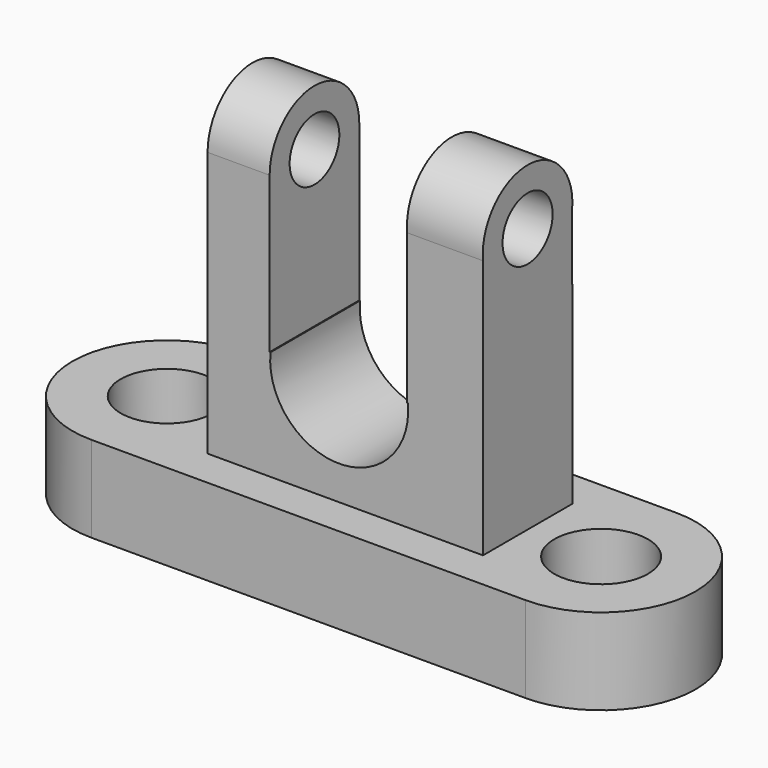
from build123d import *

# Parameters (mm, degrees)
F0_R     = 13.6198201134
F0_R_2   = 13.8204624453
F1_DEPTH = 25.4
F3_DEPTH = 16.51
F4_R     = 9.1529854274
F5_DEPTH = 18.288
F6_R     = 9.2248596532
F7_DEPTH = 22.352


# Not quite as in the source:
# - a feature names something its author has since deleted; it is built from what else it names


with BuildPart() as f1:
    # F0 (on Top) → F1 (new body)
    with BuildSketch(Plane.XY):
        with BuildLine():
            Line((-63.97113204, -27.8375800699), (63.97113204, -27.8375800699))
            ThreePointArc((63.97113204, -27.8375800699), (91.8087121099, 0), (63.97113204, 27.8375800699))
            Line((63.97113204, 27.8375800699), (-63.97113204, 27.8375800699))
            ThreePointArc((-63.97113204, 27.8375800699), (-91.8087121099, 0), (-63.97113204, -27.8375800699))
        make_face()
        with Locations((-63.97113204, 0)):
            Circle(F0_R, mode=Mode.SUBTRACT)
        with Locations((63.97113204, 0)):
            Circle(F0_R_2, mode=Mode.SUBTRACT)
    extrude(amount=-F1_DEPTH)


with BuildPart() as f3:
    # F2 (on Front) → F3 (new body, symmetric)
    with BuildSketch(Plane.XZ):
        with BuildLine():
            Line((-38.7753397226, 32.2974100709), (-38.7753397226, 0))
            Line((-38.7753397226, 0), (42.3823483288, 0))
            Line((42.3823483288, 0), (42.3823483288, 32.2974100709))
            Line((42.3823483288, 32.2974100709), (20.2484317124, 32.2974100709))
            ThreePointArc((20.2484317124, 32.2974100709), (0, 10.0047543374), (-20.2484317124, 32.2974100709))
            Line((-20.2484317124, 32.2974100709), (-38.7753397226, 32.2974100709))
        make_face()
    extrude(amount=F3_DEPTH, both=True)

    # F4 (on face) → F5 (join)
    with BuildSketch(Plane(origin=(-38.7753397226, 0, 0), x_dir=(0, -1, 0), z_dir=(-1, 0, 0))):
        with BuildLine():
            Line((-16.51, 78.1664475799), (-16.51, 56.965649128))
            Line((-16.51, 56.965649128), (-16.51, 32.2974100709))
            Line((-16.51, 32.2974100709), (16.51, 32.2974100709))
            Line((16.51, 32.2974100709), (16.51, 56.965649128))
            Line((16.51, 56.965649128), (16.51, 78.1664475799))
            ThreePointArc((16.51, 78.1664475799), (0, 94.6764475799), (-16.51, 78.1664475799))
        make_face()
        with Locations((0, 78.1664475799)):
            Circle(F4_R, mode=Mode.SUBTRACT)
    extrude(amount=-F5_DEPTH)

    # F6 (on face) → F7 (join)
    with BuildSketch(Plane.YZ.offset(42.3823483288)):
        with BuildLine():
            Line((-16.51, 76.4174684882), (-16.51, 56.965649128))
            Line((-16.51, 56.965649128), (-16.51, 32.2974100709))
            Line((-16.51, 32.2974100709), (16.51, 32.2974100709))
            Line((16.51, 32.2974100709), (16.51, 56.965649128))
            Line((16.51, 56.965649128), (16.3297262043, 56.965649128))
            Line((16.3297262043, 56.965649128), (16.3297262043, 76.4174684882))
            ThreePointArc((16.3297262043, 76.4174684882), (-0.0901368979, 94.5924619413), (-16.51, 76.4174684882))
        make_face()
        with Locations((-0.0901368979, 78.0878537591)):
            Circle(F6_R, mode=Mode.SUBTRACT)
    extrude(amount=-F7_DEPTH)


solid = Compound([f1.part, f3.part])
